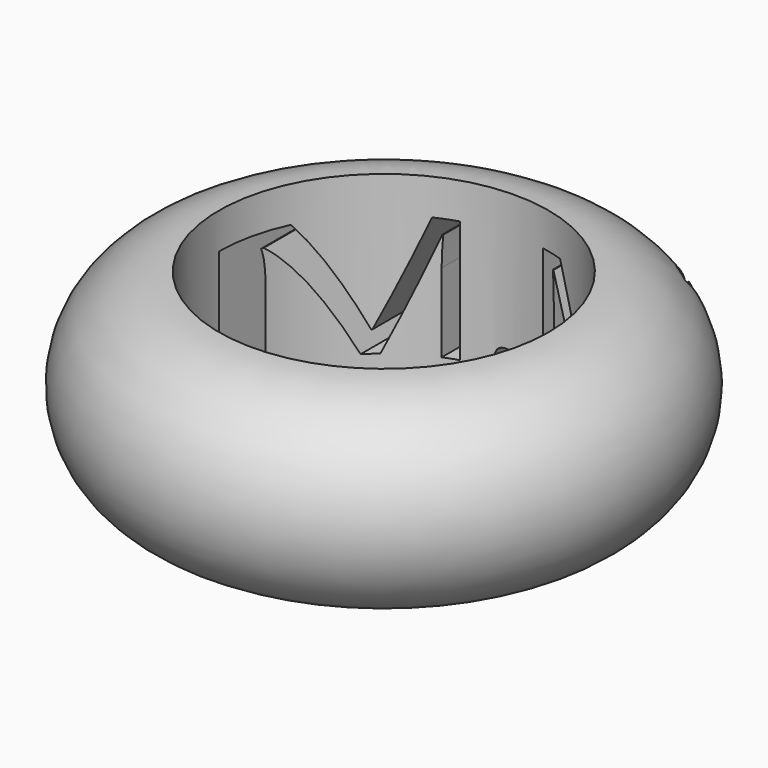
from build123d import *

# Parameters (mm, degrees)
F2_TEXT_SIZE = 9.8595195191
F3_DEPTH     = 25.4


# Not quite as in the source:
# - Text() gives the source's letters only with a copy of the font that has no kerning and outlines rounded to 1/6400 em; it was checked with that copy


with BuildPart() as f1:
    # F0 (on Front) → F1 (revolve)
    with BuildSketch(Plane.XZ):
        with BuildLine():
            Line((9.4996, 5.715), (9.4996, -5.715))
            ThreePointArc((9.4996, -5.715), (15.2146, 0), (9.4996, 5.715))
        make_face()
    revolve(axis=Axis((0, 0, 5.4870629683), (0, 0, 1)))

    # F2 (on Front) → F3 (cut)
    with BuildSketch(Plane.XZ):
        with Locations((-10.7961734757, -3.4015341662)):
            Text('M.M', F2_TEXT_SIZE, font='Open Sans', text_align=(TextAlign.LEFT, TextAlign.BOTTOM))
    extrude(amount=-F3_DEPTH, mode=Mode.SUBTRACT)


solid = f1.part
